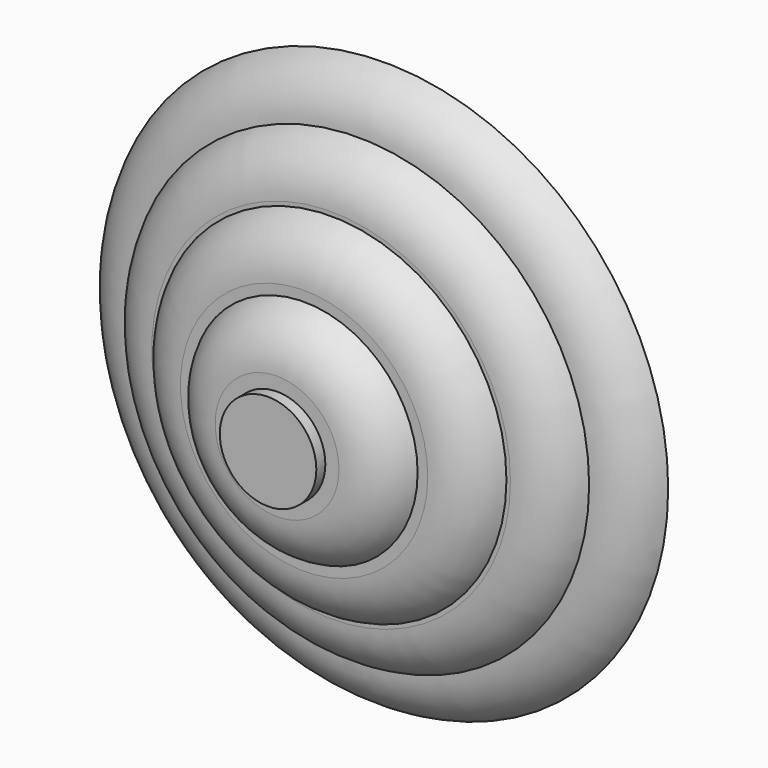
from build123d import *

# Parameters (mm, degrees)
F0_R     = 25.1181711361
F0_R_2   = 20.4995111856
F1_DEPTH = 3
F0_R_3   = 15.560509686
F2_DEPTH = 6
F0_R_4   = 10.0770984701
F3_DEPTH = 9
F0_R_5   = 4.2848341216
F4_DEPTH = 12
F0_R_6   = 1.2539122761
F5_DEPTH = 13
F6_DEPTH = 13
F7_DEPTH = 15


# Not quite as in the source:
# - a fillet or chamfer that OpenCascade refuses, or shapes differently, is made with other operations: its cross-section is extruded or revolved along the edge and cut away or added


with BuildPart() as f1:
    # F0 (on Front) → F1 (new body)
    with BuildSketch(Plane.XZ):
        Circle(F0_R)
        Circle(F0_R_2, mode=Mode.SUBTRACT)
    extrude(amount=F1_DEPTH)

    # F0 (on Front) → F2 (join)
    with BuildSketch(Plane.XZ):
        Circle(F0_R_2)
        Circle(F0_R_3, mode=Mode.SUBTRACT)
    extrude(amount=F2_DEPTH)

    # F0 (on Front) → F3 (join)
    with BuildSketch(Plane.XZ):
        Circle(F0_R_3)
        Circle(F0_R_4, mode=Mode.SUBTRACT)
    extrude(amount=F3_DEPTH)

    # F0 (on Front) → F4 (join)
    with BuildSketch(Plane.XZ):
        Circle(F0_R_4)
        Circle(F0_R_5, mode=Mode.SUBTRACT)
    extrude(amount=F4_DEPTH)

    # F0 (on Front) → F5 (join)
    with BuildSketch(Plane.XZ):
        Circle(F0_R_5)
        Circle(F0_R_6, mode=Mode.SUBTRACT)
    extrude(amount=F5_DEPTH)

    # F0 (on Front) → F6 (join)
    with BuildSketch(Plane.XZ):
        Circle(F0_R_6)
    extrude(amount=F6_DEPTH)

    # F0 (on Front) → F7 (join)
    with BuildSketch(Plane.XZ):
        Circle(F0_R_6)
    extrude(amount=-F7_DEPTH)

    # F8: fillet of radius 5 on 4 edges, made by hand

    # F8_s1 → F8_t2 (revolve, cut)
    with BuildSketch(Plane.XY):
        with BuildLine():
            ThreePointArc((25.1181711361, 0), (23.2742082286, -2.1833001327), (20.5355954411, -3))
            Line((20.5355954411, -3), (25.1181711361, -3))
            Line((25.1181711361, -3), (25.1181711361, 0))
        make_face()
    revolve(axis=Axis((0, -3, 0), (0, -1, 0)), mode=Mode.SUBTRACT)

    # F8_s3 → F8_t4 (revolve, cut)
    with BuildSketch(Plane.XY):
        with BuildLine():
            ThreePointArc((20.4995111856, -3), (18.6555482782, -5.1833001327), (15.9169354907, -6))
            Line((15.9169354907, -6), (20.4995111856, -6))
            Line((20.4995111856, -6), (20.4995111856, -3))
        make_face()
    revolve(axis=Axis((0, -6, 0), (0, -1, 0)), mode=Mode.SUBTRACT)

    # F8_s5 → F8_t6 (revolve, cut)
    with BuildSketch(Plane.XY):
        with BuildLine():
            ThreePointArc((15.560509686, -6), (13.7165467785, -8.1833001327), (10.977933991, -9))
            Line((10.977933991, -9), (15.560509686, -9))
            Line((15.560509686, -9), (15.560509686, -6))
        make_face()
    revolve(axis=Axis((0, -9, 0), (0, -1, 0)), mode=Mode.SUBTRACT)

    # F8_s7 → F8_t8 (revolve, cut)
    with BuildSketch(Plane.XY):
        with BuildLine():
            ThreePointArc((10.0770984701, -9), (8.2331355627, -11.1833001327), (5.4945227752, -12))
            Line((5.4945227752, -12), (10.0770984701, -12))
            Line((10.0770984701, -12), (10.0770984701, -9))
        make_face()
    revolve(axis=Axis((0, -12, 0), (0, -1, 0)), mode=Mode.SUBTRACT)


solid = f1.part
